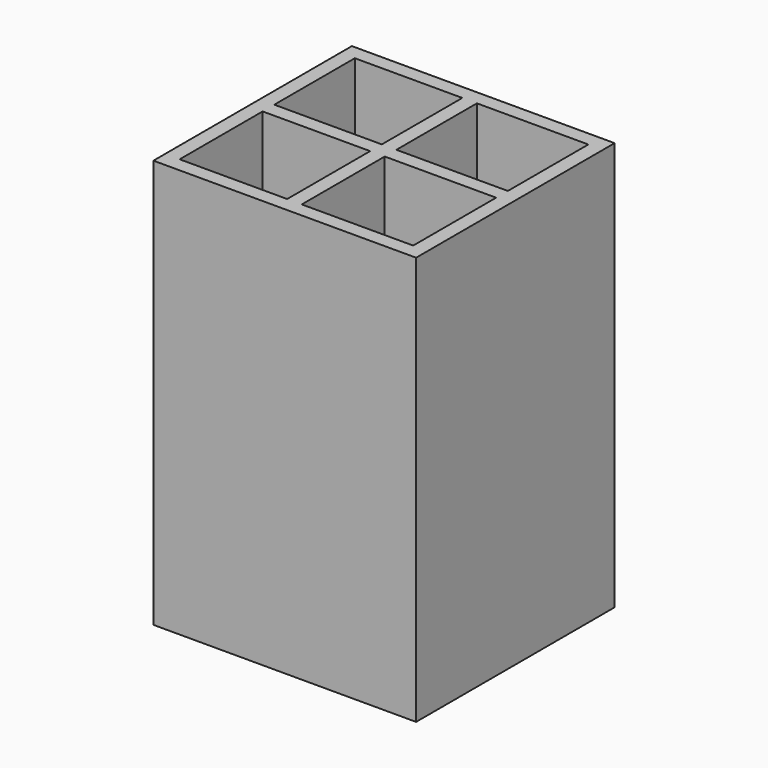
from build123d import *

# Parameters (mm, degrees)
F0_W      = 57.15
F0_H      = 88.9
F1_DEPTH  = 3.175
F2_W      = 3.175
F2_H      = 88.9
F3_DEPTH  = 50.8
F4_W      = 3.175
F4_H      = 88.9
F5_DEPTH  = 50.8
F6_W      = 53.0491641998
F6_H      = 88.9
F7_DEPTH  = 3.175
F8_W      = 50.8
F8_H      = 47.625
F9_DEPTH  = 3.175
F11_W     = 50.8
F11_H     = 47.625
F12_DEPTH = 3.175
F13_W     = 3.175
F13_H     = 85.725
F14_DEPTH = 50.8
F15_W     = 3.175
F15_H     = 85.725
F16_DEPTH = 50.8


with BuildPart() as f1:
    # F0 (on Front) → F1 (new body)
    with BuildSketch(Plane.XZ):
        with Locations((6.8577993661, 8.5990129304)):
            Rectangle(F0_W, F0_H)
    extrude(amount=F1_DEPTH)

    # F2 (on face) → F3 (join)
    with BuildSketch(Plane.XZ.offset(3.175)):
        with Locations((-20.1297006339, 8.5990129304)):
            Rectangle(F2_W, F2_H)
    extrude(amount=F3_DEPTH)

    # F4 (on face) → F5 (join)
    with BuildSketch(Plane.XZ.offset(3.175)):
        with Locations((33.8452993661, 8.5990129304)):
            Rectangle(F4_W, F4_H)
    extrude(amount=F5_DEPTH)

    # F6 (on face) → F7 (join)
    with BuildSketch(Plane.XZ.offset(53.975)):
        with Locations((5.7332172662, 8.5990129304)):
            Rectangle(F6_W, F6_H)
    extrude(amount=-F7_DEPTH)

    # F11 (on face) → F12 (join)
    with BuildSketch(Plane(origin=(0, 0, -35.8509870696), x_dir=(1, 0, 0), z_dir=(0, 0, -1))):
        with Locations((6.8577993661, 26.9875)):
            Rectangle(F11_W, F11_H)
    extrude(amount=-F12_DEPTH)

    # F13 (on face) → F14 (join)
    with BuildSketch(Plane.XZ.offset(3.175)):
        with Locations((6.430921746, 10.1865129304)):
            Rectangle(F13_W, F13_H)
    extrude(amount=F14_DEPTH)

    # F15 (on face) → F16 (join)
    with BuildSketch(Plane.YZ.offset(-18.5422006339)):
        with Locations((-26.6523276031, 10.1865129304)):
            Rectangle(F15_W, F15_H)
    extrude(amount=F16_DEPTH)


with BuildPart() as f9:
    # F8 (on face) → F9 (new body)
    with BuildSketch(Plane(origin=(0, 0, -35.8509870696), x_dir=(1, 0, 0), z_dir=(0, 0, -1))):
        with Locations((6.8577993661, 26.9875)):
            Rectangle(F8_W, F8_H)
    extrude(amount=-F9_DEPTH)


solid = f1.part
